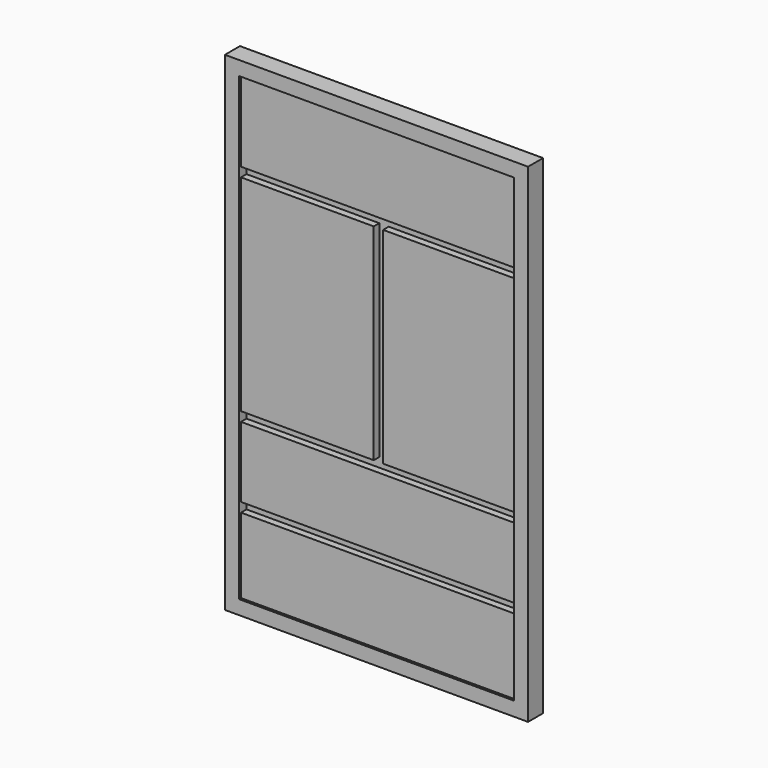
from build123d import *

# Parameters (mm, degrees)
F1_DEPTH      = 12.7
F1_DEPTH_BACK = 12.7
F0_W          = 371.475
F0_H          = 622.3
F2_DEPTH      = 9.398
F2_DEPTH_BACK = 9.398
F3_W          = 371.475
F3_H          = 12.7
F4_DEPTH      = 12.7


# Not quite as in the source:
# - a feature names something its author has since deleted; it is built from what else it names


with BuildPart() as f1:
    # F0 (on Front) → F1 (new body, two sides)
    with BuildSketch(Plane.XZ) as f1_sk:
        Polygon((263.0418609804, 506.0493900317), (634.5168609804, 506.0493900317), (653.5668609804, 525.0993900317), (243.9918609804, 525.0993900317), align=None)
        Polygon((653.5668609804, 525.0993900317), (634.5168609804, 506.0493900317), (634.5168609804, -116.2506099683), (653.5668609804, -135.3006099683), align=None)
        Polygon((653.5668609804, -135.3006099683), (634.5168609804, -116.2506099683), (263.0418609804, -116.2506099683), (243.9918609804, -135.3006099683), align=None)
        Polygon((263.0418609804, -116.2506099683), (263.0418609804, 506.0493900317), (243.9918609804, 525.0993900317), (243.9918609804, -135.3006099683), align=None)
    extrude(amount=-F1_DEPTH)
    extrude(f1_sk.sketch, amount=F1_DEPTH_BACK)

    # F0 (on Front) → F2 (join, two sides)
    with BuildSketch(Plane.XZ) as f2_sk:
        Polygon((653.5668609804, 525.0993900317), (634.5168609804, 506.0493900317), (634.5168609804, -116.2506099683), (653.5668609804, -135.3006099683), align=None)
        Polygon((263.0418609804, 506.0493900317), (634.5168609804, 506.0493900317), (653.5668609804, 525.0993900317), (243.9918609804, 525.0993900317), align=None)
        Polygon((653.5668609804, -135.3006099683), (634.5168609804, -116.2506099683), (263.0418609804, -116.2506099683), (243.9918609804, -135.3006099683), align=None)
        with Locations((448.7793609804, 194.8993900317)):
            Rectangle(F0_W, F0_H)
        Polygon((263.0418609804, -116.2506099683), (263.0418609804, 506.0493900317), (243.9918609804, 525.0993900317), (243.9918609804, -135.3006099683), align=None)
    extrude(amount=-F2_DEPTH)
    extrude(f2_sk.sketch, amount=F2_DEPTH_BACK)

    # F3 (on face) → F4 (cut)
    with BuildSketch(Plane.XZ):
        Polygon((455.1293609804, 105.9993900317), (455.1293609804, 384.1293900317), (634.5168609804, 384.1293900317), (634.5168609804, 396.8293900317), (263.0418609804, 396.8293900317), (263.0418609804, 384.1293900317), (442.4293609804, 384.1293900317), (442.4293609804, 105.9993900317), (263.0418609804, 105.9993900317), (263.0418609804, 93.2993900317), (634.5168609804, 93.2993900317), (634.5168609804, 105.9993900317), align=None)
        with Locations((448.7793609804, -8.3006099683)):
            Rectangle(F3_W, F3_H)
    extrude(amount=F4_DEPTH, mode=Mode.SUBTRACT)


solid = f1.part
